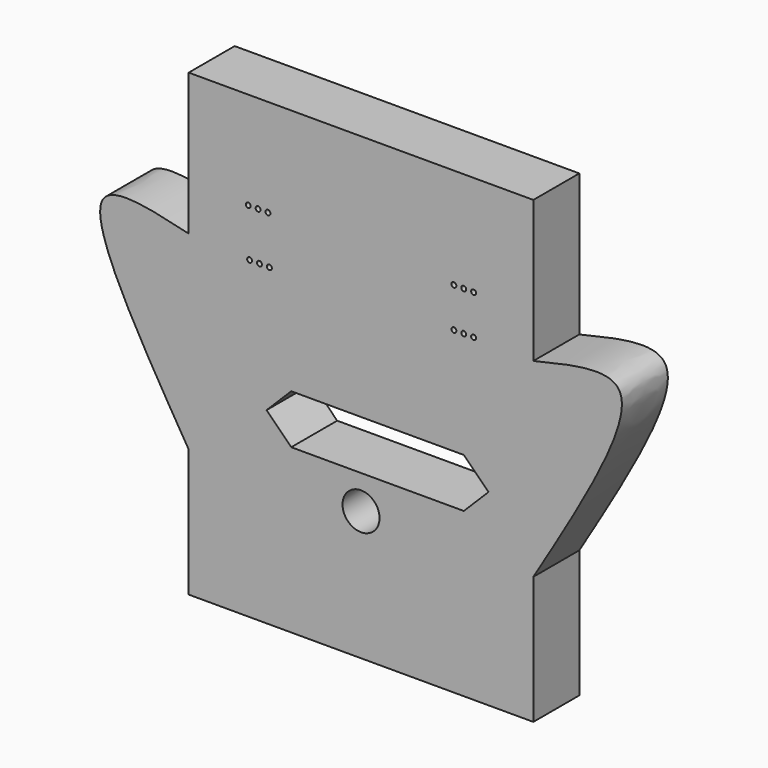
from build123d import *

# Parameters (mm, degrees)
F0_R     = 8.047855898
F0_R_2   = 1.0743657774
F1_DEPTH = 25


# Not quite as in the source:
# - the program builds the solid bodies; features that only make, move or delete a surface that nothing else refers to are left out


with BuildPart() as f1:
    # F0 (on Front) → F1 (new body)
    with BuildSketch(Plane.XZ):
        Polygon((75, 46.0328937352), (75, 107.7262044382), (-75, 107.7262044382), (-75, 46.0328937352), (-75, -36.6851300407), (-75, -92.2737955618), (75, -92.2737955618), (75, -36.6851300407), align=None)
        with Locations((0, -35.9561647287)):
            Circle(F0_R, mode=Mode.SUBTRACT)
        Polygon((44.7407775558, -21.2889015805), (-30.3720422538, -21.2889015805), (-41.1018976561, -10.5590461782), (-30.3720422538, 0.1708092241), (44.7407775558, 0.1708092241), (55.4706329581, -10.5590461782), align=None, mode=Mode.SUBTRACT)
        with Locations((-48.4804458196, 44.5564172655)):
            Circle(F0_R_2, mode=Mode.SUBTRACT)
        with Locations((-44.1829827099, 44.5564172655)):
            Circle(F0_R_2, mode=Mode.SUBTRACT)
        with Locations((-39.8855196001, 44.5564172655)):
            Circle(F0_R_2, mode=Mode.SUBTRACT)
        with Locations((-49.0825107104, 65.3187614809)):
            Circle(F0_R_2, mode=Mode.SUBTRACT)
        with Locations((-44.7850476006, 65.3187614809)):
            Circle(F0_R_2, mode=Mode.SUBTRACT)
        with Locations((-40.4875844908, 65.3187614809)):
            Circle(F0_R_2, mode=Mode.SUBTRACT)
        with Locations((40.4036690891, 46.6322604282)):
            Circle(F0_R_2, mode=Mode.SUBTRACT)
        with Locations((44.7011321989, 46.6322604282)):
            Circle(F0_R_2, mode=Mode.SUBTRACT)
        with Locations((48.9985953086, 46.6322604282)):
            Circle(F0_R_2, mode=Mode.SUBTRACT)
        with Locations((40.4036690891, 63.9077951499)):
            Circle(F0_R_2, mode=Mode.SUBTRACT)
        with Locations((44.7011321989, 63.9077951499)):
            Circle(F0_R_2, mode=Mode.SUBTRACT)
        with Locations((48.9985953086, 63.9077951499)):
            Circle(F0_R_2, mode=Mode.SUBTRACT)
        with BuildLine():
            add(Edge.make_bspline(
                [(75, 46.0328937352), (91.3344780181, 49.9824236443), (133.3315352118, 60.1369344463), (97.1245297955, 0.0384474003), (75, -36.6851300407)],
                knots=[0, 0, 0, 0, 0.3889433953, 1, 1, 1, 1], degree=3))
            Line((75, 46.0328937352), (75, -36.6851300407))
        make_face()
        with BuildLine():
            Line((-75, -36.6851300407), (-75, 46.0328937352))
            add(Edge.make_bspline(
                [(-75, 46.0328937352), (-91.3344780181, 49.9824236443), (-133.3315352118, 60.1369344463), (-97.1245297955, 0.0384474003), (-75, -36.6851300407)],
                knots=[0, 0, 0, 0, 0.3889433953, 1, 1, 1, 1], degree=3))
        make_face()
    extrude(amount=F1_DEPTH)


solid = f1.part
